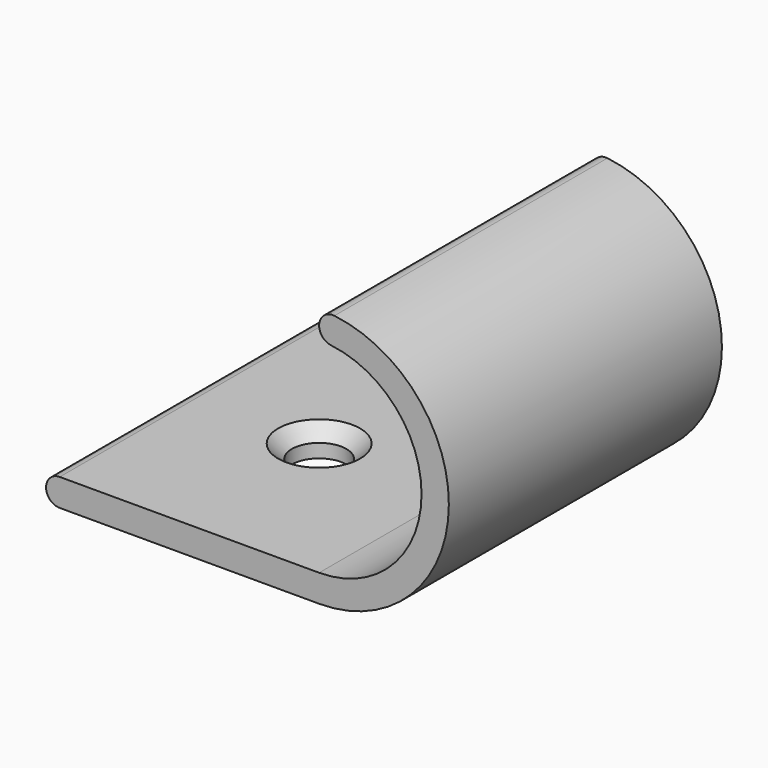
from build123d import *

# Parameters (mm, degrees)
F1_DEPTH = 12.5
F2_R     = 2
F3_DEPTH = 25
F4_SIZE  = 1
F5_R     = 0.99999


# Not quite as in the source:
# - a fillet or chamfer is up to 0.001 mm smaller than in the source, because OpenCascade refuses the exact size


with BuildPart() as f1:
    # F0 (on Front) → F1 (new body, symmetric)
    with BuildSketch(Plane.XZ):
        with BuildLine():
            ThreePointArc((10, 16), (17.5, 8.5), (10, 1))
            Line((10, 1), (-10, 1))
            Line((-10, 1), (-10, -1))
            Line((-10, -1), (10, -1))
            ThreePointArc((10, -1), (19.5, 8.5), (10, 18))
            Line((10, 18), (10, 16))
        make_face()
    extrude(amount=F1_DEPTH, both=True)

    # F2 (on face) → F3 (cut)
    with BuildSketch(Plane(origin=(0, 0, -1), x_dir=(1, 0, 0), z_dir=(0, 0, -1))):
        Circle(F2_R)
    extrude(amount=-F3_DEPTH, mode=Mode.SUBTRACT)

    # F4
    f4_edges = [f1.edges().sort_by_distance(p)[0] for p in [
        (-2, 0, 1),
    ]]
    chamfer(f4_edges, length=F4_SIZE)

    # F5 (radius 1 in the source; OpenCascade refuses exactly that, so slightly less here)
    f5_edges = [f1.edges().sort_by_distance(p)[0] for p in [
        (10, 0, 18),
        (10, 0, 16),
        (-10, 0, 1),
        (-10, 0, -1),
    ]]
    fillet(f5_edges, radius=F5_R)


solid = f1.part
